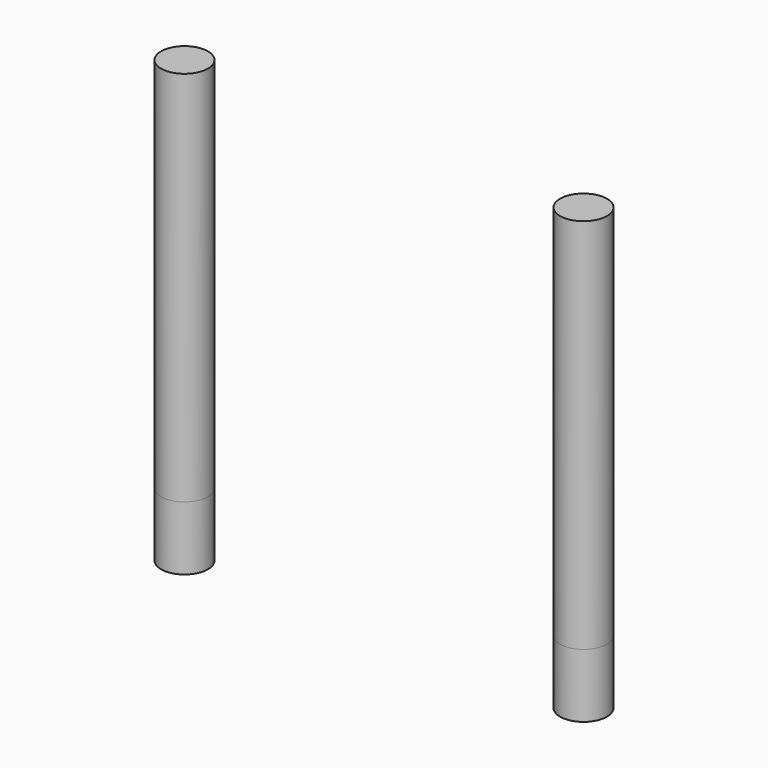
from build123d import *

# Parameters (mm, degrees)
F0_R     = 9.3327528448
F2_DEPTH = 25.4
F3_DEPTH = 150


# Not quite as in the source:
# - the program builds the solid bodies; features that only make, move or delete a surface that nothing else refers to are left out


with BuildPart() as f2:
    # F0 (on Top) → F2 (new body)
    with BuildSketch(Plane.XY):
        with Locations((-79.3886129565, 0)):
            Circle(F0_R)
    extrude(amount=F2_DEPTH)


with BuildPart() as f2b:
    # F0 (on Top) → F2, piece 2 (new body)
    with BuildSketch(Plane.XY):
        with Locations((79.3886129565, 0)):
            Circle(F0_R)
    extrude(amount=F2_DEPTH)


with BuildPart() as f3:
    # F3 (new): a face of the model
    f3_faces = [f2.part.faces().sort_by_distance(p)[0] for p in [
        (-79.3886129565, 0, 25.4),
    ]]
    extrude(f3_faces, amount=F3_DEPTH)


with BuildPart() as f3b:
    # F3#2 (new): a face of the model
    f3_2_faces = [f2b.part.faces().sort_by_distance(p)[0] for p in [
        (79.3886129565, 0, 25.4),
    ]]
    extrude(f3_2_faces, amount=F3_DEPTH)


solid = Compound([f2.part, f2b.part, f3.part, f3b.part])
